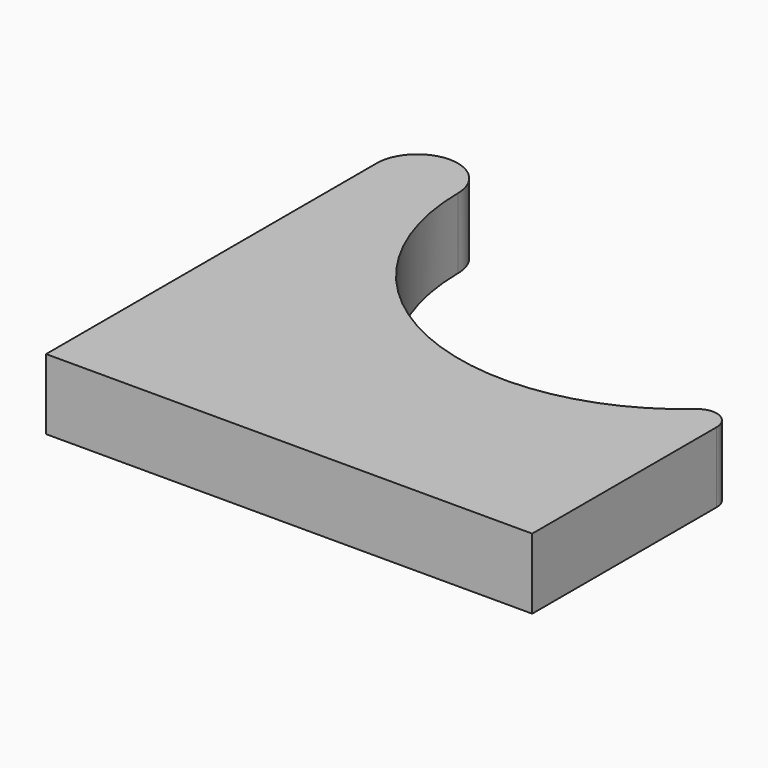
from build123d import *

# Parameters (mm, degrees)
F1_DEPTH = 5
F3_DEPTH = 5


# Not quite as in the source:
# - ends of sketch curves that miss each other by under 0.0002 mm in the source are joined
# - a feature names something its author has since deleted; it is built from what else it names


with BuildPart() as f1:
    # F0 (on Top) → F1 (new body)
    with BuildSketch(Plane.XY):
        with BuildLine():
            Line((0, 29.2999204248), (0, 0))
            Line((0, 0), (34.4714387385, 0))
            Line((34.4714387385, 0), (34.4714387385, 16.3473710418))
            ThreePointArc((34.4714387385, 16.3473710418), (32.5790927131, 15.1300794804), (32.2559916738, 17.3568210333))
            ThreePointArc((32.2559916738, 17.3568210333), (15.182844974, 14.8438668457), (5.7578901922, 29.2999210911))
            ThreePointArc((5.7578901922, 29.2999210911), (2.8789043427, 26.4210160822), (0, 29.2999204248))
        make_face()
        with BuildLine():
            ThreePointArc((5.7577396052, 29.3198639813), (2.8689325046, 32.1788074974), (0, 29.2999204248))
            ThreePointArc((0, 29.2999204248), (2.8789043427, 26.4210160822), (5.7578086853, 29.2999204248))
            ThreePointArc((5.7578086853, 29.2999204248), (5.7578117914, 29.3098925127), (5.7577396052, 29.3198639813))
        make_face()
        with BuildLine():
            ThreePointArc((32.2559916738, 17.3568210333), (32.5790927131, 15.1300794804), (34.4714387385, 16.3473710418))
            ThreePointArc((34.4714387385, 16.3473710418), (33.6883902233, 17.5646626032), (32.2559916738, 17.3568210333))
        make_face()
    extrude(amount=F1_DEPTH)

    # F2 (on face) → F3 (join)
    with BuildSketch(Plane.XY.offset(5)):
        with BuildLine():
            ThreePointArc((34.4714387385, 16.3473710418), (33.6883902233, 17.5646626032), (32.2559916738, 17.3568210333))
            ThreePointArc((32.2559916738, 17.3568210333), (15.182844974, 14.8438668457), (5.7578901922, 29.2999210911))
            ThreePointArc((5.7578901922, 29.2999210911), (5.757811792, 29.3098923335), (5.7577396052, 29.3198639813))
            ThreePointArc((5.7577396052, 29.3198639813), (2.8689325046, 32.1788074974), (0, 29.2999204248))
            Line((0, 29.2999204248), (0, 0))
            Line((0, 0), (34.4714387385, 0))
            Line((34.4714387385, 0), (34.4714387385, 16.3473710418))
        make_face()
    extrude(amount=-F3_DEPTH)


solid = f1.part
